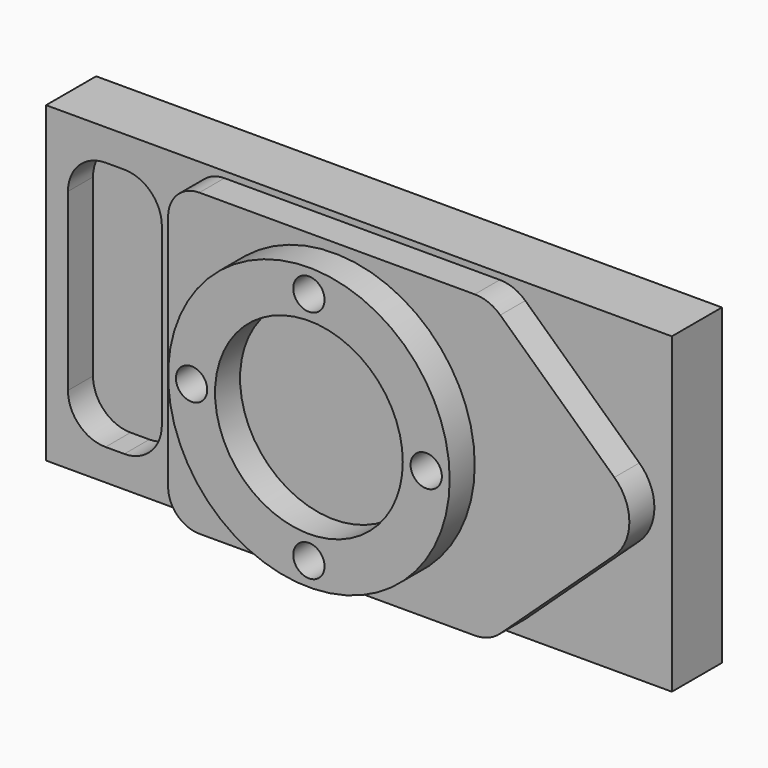
from build123d import *

# Parameters (mm, degrees)
F0_W     = 200
F0_H     = 100
F1_DEPTH = 20
F3_DEPTH = 10
F5_DEPTH = 10
F6_R     = 45
F6_R_2   = 30
F7_DEPTH = 10
F9_D     = 10
F9_DEPTH = 25
F9_TIP   = 3.0043030951


with BuildPart() as f1:
    # F0 (on Front) → F1 (new body)
    with BuildSketch(Plane.XZ):
        Rectangle(F0_W, F0_H)
    extrude(amount=F1_DEPTH)

    # F2 (on face) → F3 (cut)
    with BuildSketch(Plane.XZ.offset(20)):
        with BuildLine():
            Line((-81, -40), (-75, -40))
            ThreePointArc((-75, -40), (-66.5147186258, -36.4852813742), (-63, -28))
            Line((-63, -28), (-63, 28))
            ThreePointArc((-63, 28), (-66.5147186258, 36.4852813742), (-75, 40))
            Line((-75, 40), (-81, 40))
            ThreePointArc((-81, 40), (-89.4852813742, 36.4852813742), (-93, 28))
            Line((-93, 28), (-93, -28))
            ThreePointArc((-93, -28), (-89.4852813742, -36.4852813742), (-81, -40))
        make_face()
    extrude(amount=-F3_DEPTH, mode=Mode.SUBTRACT)

    # F4 (on face) → F5 (join)
    with BuildSketch(Plane.XZ.offset(20)):
        with BuildLine():
            ThreePointArc((-43, 48), (-50.0710678119, 45.0710678119), (-53, 38))
            Line((-53, 38), (-53, -38))
            ThreePointArc((-53, -38), (-50.0710678119, -45.0710678119), (-43, -48))
            Line((-43, -48), (45, -48))
            ThreePointArc((45, -48), (49.38178046, -47.171392035), (53.1584312217, -44.8))
            Line((53.1584312217, -44.8), (89.6164207439, -11))
            ThreePointArc((89.6164207439, -11), (94.4183817168, 0), (89.6164207439, 11))
            Line((89.6164207439, 11), (53.1584312217, 44.8))
            ThreePointArc((53.1584312217, 44.8), (49.38178046, 47.171392035), (45, 48))
            Line((45, 48), (-43, 48))
        make_face()
    extrude(amount=F5_DEPTH)

    # F6 (on face) → F7 (join)
    with BuildSketch(Plane.XZ.offset(30)):
        Circle(F6_R)
        Circle(F6_R_2, mode=Mode.SUBTRACT)
    extrude(amount=F7_DEPTH)

    # F9
    with Locations(Plane.XZ.offset(40)):
        with Locations((-37.5, 0), (0, 37.5), (37.5, 0), (0, -37.5)):
            Hole(F9_D / 2, depth=F9_DEPTH)
            with Locations((0, 0, -(F9_DEPTH + F9_TIP / 2))):  # 118° drill point
                Cone(0, F9_D / 2, F9_TIP, mode=Mode.SUBTRACT)


solid = f1.part
